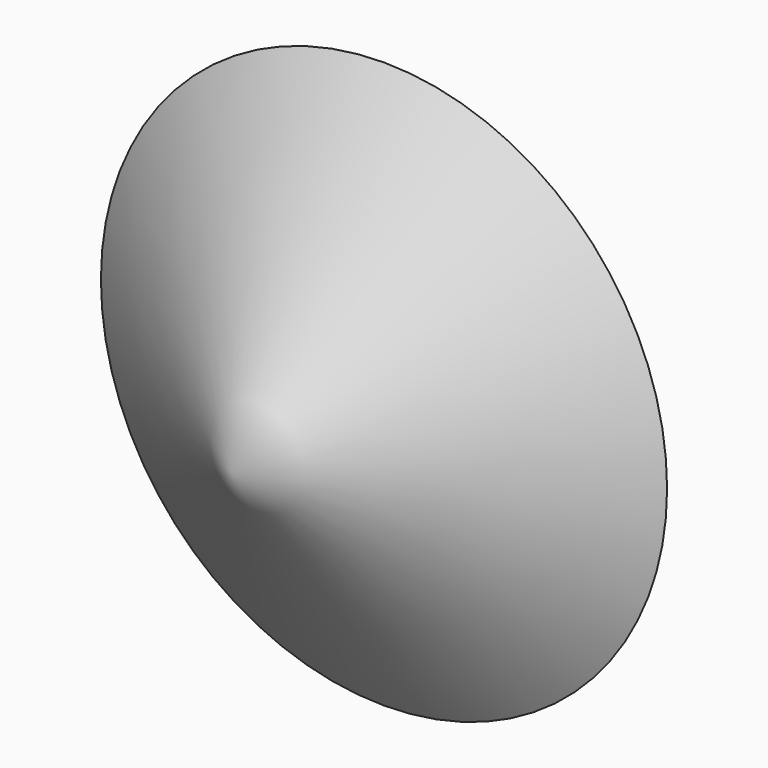
from build123d import *

# Parameters (mm, degrees)
F0_R = 23.5579264322


# Not quite as in the source:
# - an extrude whose draft closes it to a point is written as a loft to that point


with BuildPart() as f1:
    # F0 (on Front) → F1 section 0
    with BuildSketch(Plane.XZ, mode=Mode.PRIVATE) as f1_s0:
        Circle(F0_R)
    loft([f1_s0.sketch, Vertex(0, -15.8900220177, 0)], ruled=True)

    # F2: F1 across plane


with BuildPart() as f1_1:
    add(f1.part)
    add(f1.part.mirror(Plane.XZ))


solid = f1_1.part
